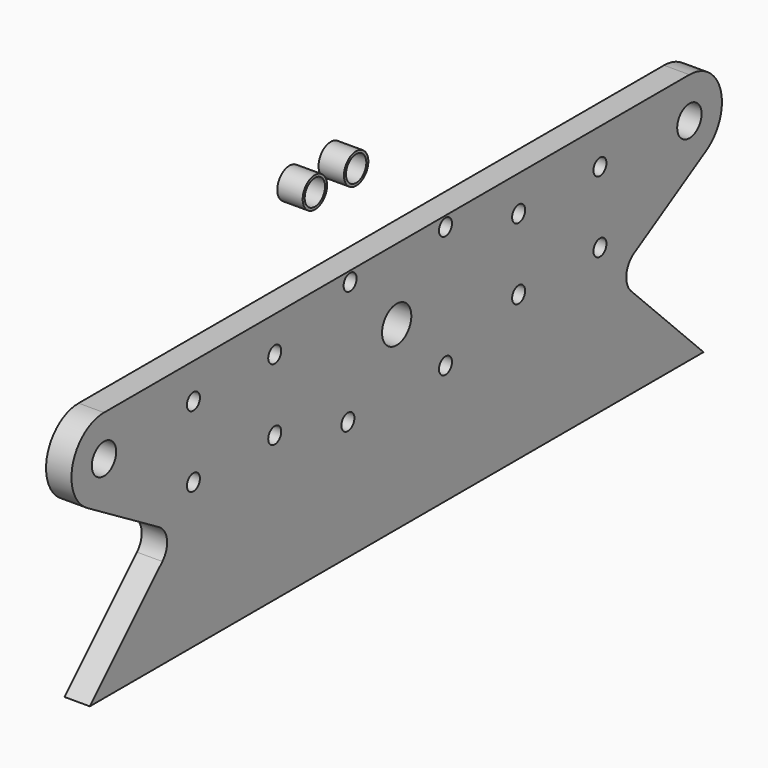
from build123d import *

# Parameters (mm, degrees)
F0_W     = 540
F0_H     = 140
F0_R     = 8
F0_R_2   = 18
F0_R_3   = 15
F1_DEPTH = 25
F2_R     = 15
F2_R_2   = 12.5
F3_DEPTH = 25
F6_R     = 20


# Not quite as in the source:
# - a feature names something its author has since deleted; it is built from what else it names


with BuildPart() as f1:
    # F0 (on Right) → F1 (new body)
    with BuildSketch(Plane.YZ):
        Rectangle(F0_W, F0_H)
        with Locations((-60, -60)):
            Circle(F0_R, mode=Mode.SUBTRACT)
        with Locations((60, -60)):
            Circle(F0_R, mode=Mode.SUBTRACT)
        with Locations((-250, -35)):
            Circle(F0_R, mode=Mode.SUBTRACT)
        with Locations((-150, -35)):
            Circle(F0_R, mode=Mode.SUBTRACT)
        with Locations((-250, 35)):
            Circle(F0_R, mode=Mode.SUBTRACT)
        with Locations((-150, 35)):
            Circle(F0_R, mode=Mode.SUBTRACT)
        with Locations((-57.3049411178, 60)):
            Circle(F0_R, mode=Mode.SUBTRACT)
        with Locations((150, -35)):
            Circle(F0_R, mode=Mode.SUBTRACT)
        Circle(F0_R_2, mode=Mode.SUBTRACT)
        with Locations((250, -35)):
            Circle(F0_R, mode=Mode.SUBTRACT)
        with Locations((150, 35)):
            Circle(F0_R, mode=Mode.SUBTRACT)
        with Locations((60, 60)):
            Circle(F0_R, mode=Mode.SUBTRACT)
        with Locations((250, 35)):
            Circle(F0_R, mode=Mode.SUBTRACT)
        with BuildLine():
            Line((-270, -70), (-270, 70))
            Line((-270, 70), (-360, 70))
            ThreePointArc((-360, 70), (-331.7157287525, 58.2842712475), (-320, 30))
            ThreePointArc((-320, 30), (-340.2169027766, -4.7653428611), (-380.4314532125, -4.3883078913))
            Line((-380.4314532125, -4.3883078913), (-270, -70))
        make_face()
        with BuildLine():
            Line((360, 70), (270, 70))
            Line((270, 70), (270, -70))
            Line((270, -70), (380.4314532125, -4.3883078913))
            ThreePointArc((380.4314532125, -4.3883078913), (321.4284281131, 19.4059525122), (360, 70))
        make_face()
        with BuildLine():
            ThreePointArc((-320, 30), (-331.7157287525, 58.2842712475), (-360, 70))
            ThreePointArc((-360, 70), (-398.5715718869, 40.5940474878), (-380.4314532125, -4.3883078913))
            ThreePointArc((-380.4314532125, -4.3883078913), (-340.2169027766, -4.7653428611), (-320, 30))
        make_face()
        with Locations((-360, 30)):
            Circle(F0_R_3, mode=Mode.SUBTRACT)
        with BuildLine():
            ThreePointArc((400, 30), (388.2842712475, 58.2842712475), (360, 70))
            ThreePointArc((360, 70), (321.4284281131, 19.4059525122), (380.4314532125, -4.3883078913))
            ThreePointArc((380.4314532125, -4.3883078913), (394.7653428611, 10.2169027766), (400, 30))
        make_face()
        with Locations((360, 30)):
            Circle(F0_R_3, mode=Mode.SUBTRACT)
        Polygon((270, -70), (-270, -70), (-377.3844690551, -177.3844690551), (377.3844690551, -177.3844690551), align=None)
    extrude(amount=F1_DEPTH)

    # F6
    f6_edges = [f1.edges().sort_by_distance(p)[0] for p in [
        (12.5, -270, -70),
        (12.5, 270, -70),
    ]]
    fillet(f6_edges, radius=F6_R)


with BuildPart() as f3:
    # F2 (on Right) → F3 (new body)
    with BuildSketch(Plane.YZ):
        with Locations((-213.5602489911, 155.390098691)):
            Circle(F2_R)
        with Locations((-213.5602489911, 155.390098691)):
            Circle(F2_R_2, mode=Mode.SUBTRACT)
    extrude(amount=F3_DEPTH)


with BuildPart() as f3b:
    # F2 (on Right) → F3, piece 2 (new body)
    with BuildSketch(Plane.YZ):
        with Locations((-154.9366889584, 155.390098691)):
            Circle(F2_R)
        with Locations((-154.9366889584, 155.390098691)):
            Circle(F2_R_2, mode=Mode.SUBTRACT)
    extrude(amount=F3_DEPTH)


with BuildPart() as f3c:
    # F2 (on Right) → F3, piece 3 (new body)
    with BuildSketch(Plane.YZ):
        with Locations((-100.630173799, 155.390098691)):
            Circle(F2_R)
        with Locations((-100.630173799, 155.390098691)):
            Circle(F2_R_2, mode=Mode.SUBTRACT)
    extrude(amount=F3_DEPTH)


with BuildPart() as f3d:
    # F2 (on Right) → F3, piece 4 (new body)
    with BuildSketch(Plane.YZ):
        with Locations((-49.8730993964, 155.390098691)):
            Circle(F2_R)
        with Locations((-49.8730993964, 155.390098691)):
            Circle(F2_R_2, mode=Mode.SUBTRACT)
    extrude(amount=F3_DEPTH)


solid = Compound([f1.part, f3c.part, f3d.part])
